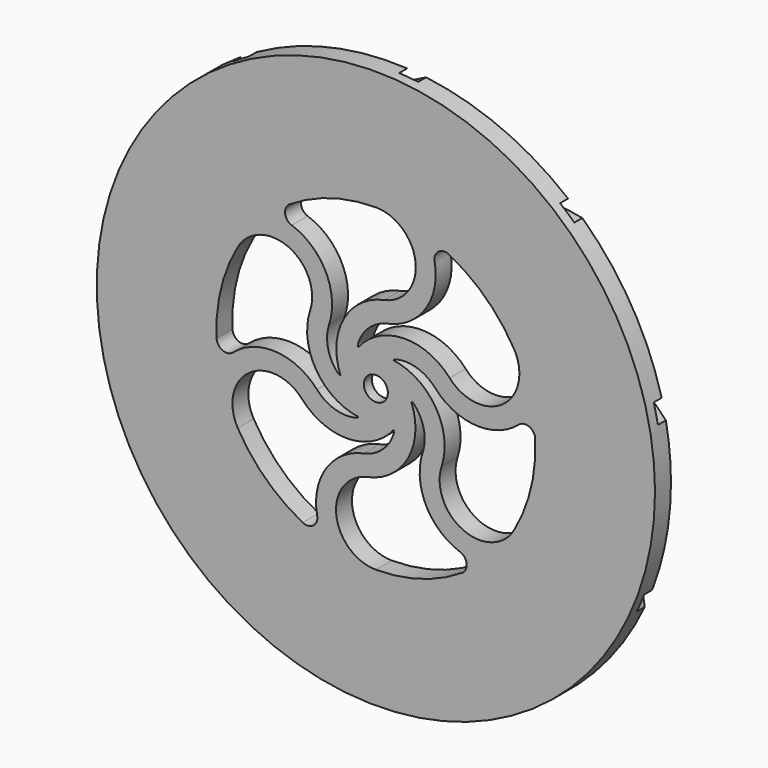
from build123d import *

# Parameters (mm, degrees)
F0_R           = 88.9
F1_DEPTH       = 6.35
F2_R           = 57.15
F2_R_2         = 53.975
F3_DEPTH       = 41.275
F5_DEPTH       = 41.275
F6_R           = 9.525
F6_R_2         = 3.81
F7_DEPTH       = 41.275
F8_R           = 3.81
F9_DEPTH       = 25.4
F10_R          = 2.54
F11_R          = 53.975
F12_DEPTH      = 41.2760001
F12_DEPTH_BACK = 3.175
F13_R          = 9.525
F13_R_2        = 3.81
F14_DEPTH      = 41.276
F14_DEPTH_BACK = 3.175


with BuildPart() as f1:
    # F0 (on Front) → F1 (new body)
    with BuildSketch(Plane.XZ):
        Circle(F0_R)
    extrude(amount=F1_DEPTH)

    # F2 (on face) → F3 (join)
    with BuildSketch(Plane.XZ.offset(6.35)):
        Circle(F2_R)
        Circle(F2_R_2, mode=Mode.SUBTRACT)
    extrude(amount=F3_DEPTH)

    # F4 (on face) → F5 (join, through all)
    with BuildSketch(Plane.XZ.offset(6.35)):
        with BuildLine():
            ThreePointArc((53.9069410952, -2.7096728137), (72.2551452316, -16.3352447412), (80.5410246247, -37.6344702686))
            ThreePointArc((80.5410246247, -37.6344702686), (81.7707619042, -34.8819795541), (82.9064652139, -32.0893755897))
            ThreePointArc((82.9064652139, -32.0893755897), (72.7373983183, -11.9238182989), (53.9711869017, 0.6415679441))
            ThreePointArc((53.9711869017, 0.6415679441), (53.9650843479, -1.0345512645), (53.9069410952, -2.7096728137))
        make_face()
        with BuildLine():
            ThreePointArc((45.2043371792, 29.4935336165), (68.0572563749, 29.2550181665), (87.2800442675, 16.8939004574))
            ThreePointArc((87.2800442675, 16.8939004574), (86.6570491761, 19.8435336593), (85.9344010285, 22.7703473815))
            ThreePointArc((85.9344010285, 22.7703473815), (65.8544359133, 33.10739838), (43.2865032341, 32.2425070794))
            ThreePointArc((43.2865032341, 32.2425070794), (44.2667643164, 30.8829111639), (45.2043371792, 29.4935336165))
        make_face()
        with BuildLine():
            ThreePointArc((19.2352128997, 50.4312126535), (37.863808764, 63.6708584761), (60.6810535397, 64.9693754112))
            ThreePointArc((60.6810535397, 64.9693754112), (58.4432890276, 66.9894914717), (56.1383164531, 68.9325715886))
            ThreePointArc((56.1383164531, 68.9325715886), (33.8173172993, 65.4927141568), (16.0678465853, 51.5279043928))
            ThreePointArc((16.0678465853, 51.5279043928), (17.6600448879, 51.0041511993), (19.2352128997, 50.4312126535))
        make_face()
        with BuildLine():
            ThreePointArc((-14.0811089267, 52.1058825508), (-6.7923268512, 73.7665949407), (10.9039628328, 88.2287571857))
            ThreePointArc((10.9039628328, 88.2287571857), (7.9061788848, 88.547740431), (4.8993030638, 88.7648963808))
            ThreePointArc((4.8993030638, 88.7648963808), (-11.1368671147, 72.8620391412), (-17.2881813331, 51.1313935972))
            ThreePointArc((-17.2881813331, 51.1313935972), (-15.6922114449, 51.6435390438), (-14.0811089267, 52.1058825508))
        make_face()
        with BuildLine():
            ThreePointArc((-42.0189257424, 33.8778763274), (-48.854024472, 55.6859993723), (-43.0380710641, 77.7877525005))
            ThreePointArc((-43.0380710641, 77.7877525005), (-45.6508228708, 76.2837621727), (-48.2110775747, 74.6920477634))
            ThreePointArc((-48.2110775747, 74.6920477634), (-51.837146819, 52.4005416633), (-44.0407115859, 31.2044283397))
            ThreePointArc((-44.0407115859, 31.2044283397), (-43.0505763644, 32.5568502729), (-42.0189257424, 33.8778763274))
        make_face()
        with BuildLine():
            ThreePointArc((-53.9069410952, 2.7096728137), (-72.2551452316, 16.3352447412), (-80.5410246247, 37.6344702686))
            ThreePointArc((-80.5410246247, 37.6344702686), (-81.7707619042, 34.8819795541), (-82.9064652139, 32.0893755897))
            ThreePointArc((-82.9064652139, 32.0893755897), (-72.7373983183, 11.9238182989), (-53.9711869017, -0.6415679441))
            ThreePointArc((-53.9711869017, -0.6415679441), (-53.9650843479, 1.0345512645), (-53.9069410952, 2.7096728137))
        make_face()
        with BuildLine():
            ThreePointArc((-45.2043371792, -29.4935336165), (-68.0572563749, -29.2550181665), (-87.2800442675, -16.8939004574))
            ThreePointArc((-87.2800442675, -16.8939004574), (-86.6570491761, -19.8435336593), (-85.9344010285, -22.7703473815))
            ThreePointArc((-85.9344010285, -22.7703473815), (-65.8544359133, -33.10739838), (-43.2865032341, -32.2425070794))
            ThreePointArc((-43.2865032341, -32.2425070794), (-44.2667643164, -30.8829111639), (-45.2043371792, -29.4935336165))
        make_face()
        with BuildLine():
            ThreePointArc((-19.2352128997, -50.4312126535), (-37.863808764, -63.6708584761), (-60.6810535397, -64.9693754112))
            ThreePointArc((-60.6810535397, -64.9693754112), (-58.4432890276, -66.9894914717), (-56.1383164531, -68.9325715886))
            ThreePointArc((-56.1383164531, -68.9325715886), (-33.8173172993, -65.4927141568), (-16.0678465853, -51.5279043928))
            ThreePointArc((-16.0678465853, -51.5279043928), (-17.6600448879, -51.0041511993), (-19.2352128997, -50.4312126535))
        make_face()
        with BuildLine():
            ThreePointArc((14.0811089267, -52.1058825508), (6.7923268512, -73.7665949407), (-10.9039628328, -88.2287571857))
            ThreePointArc((-10.9039628328, -88.2287571857), (-7.9061788848, -88.547740431), (-4.8993030638, -88.7648963808))
            ThreePointArc((-4.8993030638, -88.7648963808), (11.1368671147, -72.8620391412), (17.2881813331, -51.1313935972))
            ThreePointArc((17.2881813331, -51.1313935972), (15.6922114449, -51.6435390438), (14.0811089267, -52.1058825508))
        make_face()
        with BuildLine():
            ThreePointArc((42.0189257424, -33.8778763274), (48.854024472, -55.6859993723), (43.0380710641, -77.7877525005))
            ThreePointArc((43.0380710641, -77.7877525005), (45.6508228708, -76.2837621727), (48.2110775747, -74.6920477634))
            ThreePointArc((48.2110775747, -74.6920477634), (51.837146819, -52.4005416633), (44.0407115859, -31.2044283397))
            ThreePointArc((44.0407115859, -31.2044283397), (43.0505763644, -32.5568502729), (42.0189257424, -33.8778763274))
        make_face()
    extrude(amount=F5_DEPTH)

    # F6 (on face) → F7 (join, through all)
    with BuildSketch(Plane.XZ.offset(6.35)):
        Circle(F6_R)
        Circle(F6_R_2, mode=Mode.SUBTRACT)
    extrude(amount=F7_DEPTH)

    # F8 (on face) → F9 (cut)
    with BuildSketch(Plane.XZ.offset(6.35)):
        Circle(F8_R)
        with BuildLine():
            ThreePointArc((18.7012290876, 41.7285714286), (15.8576147996, 27.543553966), (3.8682590056, 19.446875))
            ThreePointArc((3.8682590056, 19.446875), (-2.091465664, 16.4126776534), (-5.6835018732, 10.7715831188))
            ThreePointArc((-5.6835018732, 10.7715831188), (-5.7538490333, 10.2503071963), (-5.6500021555, 9.7346589282))
            ThreePointArc((-5.6500021555, 9.7346589282), (8.7313709485, 16.9640191411), (23.5156008127, 10.5989512885))
            ThreePointArc((23.5156008127, 10.5989512885), (40.4349404037, 8.7570054641), (43.9940905122, 25.4))
            ThreePointArc((43.9940905122, 25.4), (35.0538695993, 36.7677334917), (23.2726406424, 45.1555555556))
            ThreePointArc((23.2726406424, 45.1555555556), (19.9136606493, 44.8737532722), (18.7012290876, 41.7285714286))
        make_face()
        with BuildLine():
            ThreePointArc((-11.2554630068, -0.025715934), (-10.3255860522, 16.0435986218), (2.5788393371, 25.6645833333))
            ThreePointArc((2.5788393371, 25.6645833333), (12.6336810088, 39.3961883222), (0, 50.8))
            ThreePointArc((0, 50.8), (-14.3148564437, 48.7414083198), (-27.4695379119, 42.7324757872))
            ThreePointArc((-27.4695379119, 42.7324757872), (-28.9049799722, 39.6826126407), (-26.787388377, 37.0600251862))
            ThreePointArc((-26.787388377, 37.0600251862), (-15.9246100453, 27.5048742428), (-14.9073582714, 13.0734480673))
            ThreePointArc((-14.9073582714, 13.0734480673), (-15.259528624, 6.3950764305), (-12.1702155565, 0.4637345547))
            ThreePointArc((-12.1702155565, 0.4637345547), (-11.7539509452, 0.1421741658), (-11.2554630068, -0.025715934))
        make_face()
        with BuildLine():
            ThreePointArc((-5.6054608513, -9.7603748622), (-19.0569570007, -0.9204205192), (-20.9367614757, 15.0656320448))
            ThreePointArc((-20.9367614757, 15.0656320448), (-27.8012593949, 30.6391828581), (-43.9940905122, 25.4))
            ThreePointArc((-43.9940905122, 25.4), (-49.368726043, 11.9736748281), (-50.7421785543, -2.4230797683))
            ThreePointArc((-50.7421785543, -2.4230797683), (-48.8186406215, -5.1911406315), (-45.4886174646, -4.6685462424))
            ThreePointArc((-45.4886174646, -4.6685462424), (-31.7822248448, -0.0386797232), (-18.775617277, -6.3734269327))
            ThreePointArc((-18.775617277, -6.3734269327), (-13.1680629599, -10.0176012229), (-6.4867136833, -10.3078485641))
            ThreePointArc((-6.4867136833, -10.3078485641), (-6.0001019119, -10.1081330305), (-5.6054608513, -9.7603748622))
        make_face()
        with BuildLine():
            ThreePointArc((5.6500021555, -9.7346589282), (-8.7313709485, -16.9640191411), (-23.5156008127, -10.5989512885))
            ThreePointArc((-23.5156008127, -10.5989512885), (-40.4349404037, -8.7570054641), (-43.9940905122, -25.4))
            ThreePointArc((-43.9940905122, -25.4), (-35.0538695993, -36.7677334917), (-23.2726406424, -45.1555555556))
            ThreePointArc((-23.2726406424, -45.1555555556), (-19.9136606493, -44.8737532722), (-18.7012290876, -41.7285714286))
            ThreePointArc((-18.7012290876, -41.7285714286), (-15.8576147996, -27.543553966), (-3.8682590056, -19.446875))
            ThreePointArc((-3.8682590056, -19.446875), (2.091465664, -16.4126776534), (5.6835018732, -10.7715831188))
            ThreePointArc((5.6835018732, -10.7715831188), (5.7538490333, -10.2503071963), (5.6500021555, -9.7346589282))
        make_face()
        with BuildLine():
            ThreePointArc((11.2554630068, 0.025715934), (10.3255860522, -16.0435986218), (-2.5788393371, -25.6645833333))
            ThreePointArc((-2.5788393371, -25.6645833333), (-12.6336810088, -39.3961883222), (0, -50.8))
            ThreePointArc((0, -50.8), (14.3148564437, -48.7414083198), (27.4695379119, -42.7324757872))
            ThreePointArc((27.4695379119, -42.7324757872), (28.9049799722, -39.6826126407), (26.787388377, -37.0600251862))
            ThreePointArc((26.787388377, -37.0600251862), (15.9246100453, -27.5048742428), (14.9073582714, -13.0734480673))
            ThreePointArc((14.9073582714, -13.0734480673), (15.259528624, -6.3950764305), (12.1702155565, -0.4637345547))
            ThreePointArc((12.1702155565, -0.4637345547), (11.7539509452, -0.1421741658), (11.2554630068, 0.025715934))
        make_face()
        with BuildLine():
            ThreePointArc((5.6054608513, 9.7603748622), (19.0569570007, 0.9204205192), (20.9367614757, -15.0656320448))
            ThreePointArc((20.9367614757, -15.0656320448), (27.8012593949, -30.6391828581), (43.9940905122, -25.4))
            ThreePointArc((43.9940905122, -25.4), (49.368726043, -11.9736748281), (50.7421785543, 2.4230797683))
            ThreePointArc((50.7421785543, 2.4230797683), (48.8186406215, 5.1911406315), (45.4886174646, 4.6685462424))
            ThreePointArc((45.4886174646, 4.6685462424), (31.7822248448, 0.0386797232), (18.775617277, 6.3734269327))
            ThreePointArc((18.775617277, 6.3734269327), (13.1680629599, 10.0176012229), (6.4867136833, 10.3078485641))
            ThreePointArc((6.4867136833, 10.3078485641), (6.0001019119, 10.1081330305), (5.6054608513, 9.7603748622))
        make_face()
    extrude(amount=-F9_DEPTH, mode=Mode.SUBTRACT)

    # F10
    f10_edges = [f1.edges().sort_by_distance(p)[0] for p in [
        (48.482356, -26.9875, 30.258613),
        (57.146896, -26.9875, -0.595661),
        (57.008616, -26.9875, -4.017481),
        (45.882689, -26.9875, -34.072002),
        (43.759523, -26.9875, -36.759035),
        (17.092855, -26.9875, -54.533997),
        (13.795779, -26.9875, -55.459886),
        (-18.225869, -26.9875, -54.165858),
        (-46.58293, -26.9875, -33.108203),
        (-21.437483, -26.9875, -52.976946),
        (-48.482356, -26.9875, -30.258613),
        (-57.008616, -26.9875, 4.017481),
        (-45.882689, -26.9875, 34.072002),
        (-57.146896, -26.9875, 0.595661),
        (-43.759523, -26.9875, 36.759035),
        (-17.092855, -26.9875, 54.533997),
        (-13.795779, -26.9875, 55.459886),
        (18.225869, -26.9875, 54.165858),
        (21.437483, -26.9875, 52.976946),
        (46.58293, -26.9875, 33.108203),
    ]]
    fillet(f10_edges, radius=F10_R)

    # F11 (on face) → F12 (cut, two sides)
    with BuildSketch(Plane.XZ.offset(6.35)) as f12_sk:
        with BuildLine():
            ThreePointArc((-10.9039628328, -88.2287571857), (-7.9061788848, -88.547740431), (-4.8993030638, -88.7648963808))
            ThreePointArc((-4.8993030638, -88.7648963808), (9.809736429, -74.9751556371), (16.9136887004, -56.1059570663))
            ThreePointArc((16.9136887004, -56.1059570663), (17.4652017585, -54.8309893719), (18.6049444803, -54.0368257847))
            ThreePointArc((18.6049444803, -54.0368257847), (30.8226195673, -48.1257584149), (41.3018706657, -39.5003541694))
            ThreePointArc((41.3018706657, -39.5003541694), (43.585469328, -38.755739099), (45.468484571, -40.2468890071))
            ThreePointArc((45.468484571, -40.2468890071), (48.7789098199, -59.3103123401), (43.0380710641, -77.7877525005))
            ThreePointArc((43.0380710641, -77.7877525005), (45.6508228708, -76.2837621727), (48.2110775747, -74.6920477634))
            ThreePointArc((48.2110775747, -74.6920477634), (52.0055342532, -54.8901566645), (46.6617157255, -35.4490559724))
            ThreePointArc((46.6617157255, -35.4490559724), (46.3584919542, -34.0934141983), (46.8137655409, -32.7809983966))
            ThreePointArc((46.8137655409, -32.7809983966), (53.2236340928, -20.8174752062), (56.6316409092, -7.6798273375))
            ThreePointArc((56.6316409092, -7.6798273375), (58.0414372783, -5.7351554754), (60.4413045354, -5.8347125026))
            ThreePointArc((60.4413045354, -5.8347125026), (74.3246939138, -19.3115268098), (80.5410246247, -37.6344702686))
            ThreePointArc((80.5410246247, -37.6344702686), (81.7707619042, -34.8819795541), (82.9064652139, -32.0893755897))
            ThreePointArc((82.9064652139, -32.0893755897), (74.3369855958, -13.8389834938), (58.5865533169, -1.2518203661))
            ThreePointArc((58.5865533169, -1.2518203661), (57.5444138906, -0.3333135935), (57.1413193063, 0.9960561938))
            ThreePointArc((57.1413193063, 0.9960561938), (55.2950293996, 14.4423759714), (50.330049164, 27.0741325096))
            ThreePointArc((50.330049164, 27.0741325096), (50.3275489442, 29.476062609), (52.3276004918, 30.8061258634))
            ThreePointArc((52.3276004918, 30.8061258634), (71.480971136, 28.0636055872), (87.2800442675, 16.8939004574))
            ThreePointArc((87.2800442675, 16.8939004574), (86.6570491761, 19.8435336593), (85.9344010285, 22.7703473815))
            ThreePointArc((85.9344010285, 22.7703473815), (68.274235062, 32.4982110017), (48.1333188249, 33.4235680723))
            ThreePointArc((48.1333188249, 33.4235680723), (46.7503255835, 33.5541014751), (45.6428312586, 34.3926511729))
            ThreePointArc((45.6428312586, 34.3926511729), (36.2456028847, 44.1857304062), (24.8040892936, 51.486693954))
            ThreePointArc((24.8040892936, 51.486693954), (23.3902474838, 53.4284266314), (24.2265316099, 55.6800712112))
            ThreePointArc((24.2265316099, 55.6800712112), (41.3339469332, 64.7193944968), (60.6810535397, 64.9693754112))
            ThreePointArc((60.6810535397, 64.9693754112), (58.4432890276, 66.9894914717), (56.1383164531, 68.9325715886))
            ThreePointArc((56.1383164531, 68.9325715886), (36.1330472904, 66.4221934682), (19.2947925332, 55.3322895323))
            ThreePointArc((19.2947925332, 55.3322895323), (18.0992018886, 54.6249902422), (16.710333013, 54.6524223671))
            ThreePointArc((16.710333013, 54.6524223671), (3.3515880106, 57.0516376435), (-10.1961896269, 56.2330882763))
            ThreePointArc((-10.1961896269, 56.2330882763), (-12.4813335101, 56.972947646), (-13.1282489173, 59.2861218524))
            ThreePointArc((-13.1282489173, 59.2861218524), (-4.601240109, 76.6545744399), (10.9039628328, 88.2287571857))
            ThreePointArc((10.9039628328, 88.2287571857), (7.9061788848, 88.547740431), (4.8993030638, 88.7648963808))
            ThreePointArc((4.8993030638, 88.7648963808), (-9.809736429, 74.9751556371), (-16.9136887004, 56.1059570663))
            ThreePointArc((-16.9136887004, 56.1059570663), (-17.4652017585, 54.8309893719), (-18.6049444803, 54.0368257847))
            ThreePointArc((-18.6049444803, 54.0368257847), (-30.8226195673, 48.1257584149), (-41.3018706657, 39.5003541694))
            ThreePointArc((-41.3018706657, 39.5003541694), (-43.585469328, 38.755739099), (-45.468484571, 40.2468890071))
            ThreePointArc((-45.468484571, 40.2468890071), (-48.7789098199, 59.3103123401), (-43.0380710641, 77.7877525005))
            ThreePointArc((-43.0380710641, 77.7877525005), (-45.6508228708, 76.2837621727), (-48.2110775747, 74.6920477634))
            ThreePointArc((-48.2110775747, 74.6920477634), (-52.0055342532, 54.8901566645), (-46.6617157255, 35.4490559724))
            ThreePointArc((-46.6617157255, 35.4490559724), (-46.3584919542, 34.0934141983), (-46.8137655409, 32.7809983966))
            ThreePointArc((-46.8137655409, 32.7809983966), (-53.2236340928, 20.8174752062), (-56.6316409092, 7.6798273375))
            ThreePointArc((-56.6316409092, 7.6798273375), (-58.0414372783, 5.7351554754), (-60.4413045354, 5.8347125026))
            ThreePointArc((-60.4413045354, 5.8347125026), (-74.3246939138, 19.3115268098), (-80.5410246247, 37.6344702686))
            ThreePointArc((-80.5410246247, 37.6344702686), (-81.7707619042, 34.8819795541), (-82.9064652139, 32.0893755897))
            ThreePointArc((-82.9064652139, 32.0893755897), (-74.3369855958, 13.8389834938), (-58.5865533169, 1.2518203661))
            ThreePointArc((-58.5865533169, 1.2518203661), (-57.5444138906, 0.3333135935), (-57.1413193063, -0.9960561938))
            ThreePointArc((-57.1413193063, -0.9960561938), (-55.2950293996, -14.4423759714), (-50.330049164, -27.0741325096))
            ThreePointArc((-50.330049164, -27.0741325096), (-50.3275489442, -29.476062609), (-52.3276004918, -30.8061258634))
            ThreePointArc((-52.3276004918, -30.8061258634), (-71.480971136, -28.0636055872), (-87.2800442675, -16.8939004574))
            ThreePointArc((-87.2800442675, -16.8939004574), (-86.6570491761, -19.8435336593), (-85.9344010285, -22.7703473815))
            ThreePointArc((-85.9344010285, -22.7703473815), (-68.274235062, -32.4982110017), (-48.1333188249, -33.4235680723))
            ThreePointArc((-48.1333188249, -33.4235680723), (-46.7503255835, -33.5541014751), (-45.6428312586, -34.3926511729))
            ThreePointArc((-45.6428312586, -34.3926511729), (-36.2456028847, -44.1857304062), (-24.8040892936, -51.486693954))
            ThreePointArc((-24.8040892936, -51.486693954), (-23.3902474838, -53.4284266314), (-24.2265316099, -55.6800712112))
            ThreePointArc((-24.2265316099, -55.6800712112), (-41.3339469332, -64.7193944968), (-60.6810535397, -64.9693754112))
            ThreePointArc((-60.6810535397, -64.9693754112), (-58.4432890276, -66.9894914717), (-56.1383164531, -68.9325715886))
            ThreePointArc((-56.1383164531, -68.9325715886), (-36.1330472904, -66.4221934682), (-19.2947925332, -55.3322895323))
            ThreePointArc((-19.2947925332, -55.3322895323), (-18.0992018886, -54.6249902422), (-16.710333013, -54.6524223671))
            ThreePointArc((-16.710333013, -54.6524223671), (-3.3515880106, -57.0516376435), (10.1961896269, -56.2330882763))
            ThreePointArc((10.1961896269, -56.2330882763), (12.4813335101, -56.972947646), (13.1282489173, -59.2861218524))
            ThreePointArc((13.1282489173, -59.2861218524), (4.601240109, -76.6545744399), (-10.9039628328, -88.2287571857))
        make_face()
        Circle(F11_R, mode=Mode.SUBTRACT)
    extrude(amount=F12_DEPTH, mode=Mode.SUBTRACT)
    extrude(f12_sk.sketch, amount=-F12_DEPTH_BACK, mode=Mode.SUBTRACT)

    # F13 (on face) → F14 (cut, two sides)
    with BuildSketch(Plane.XZ.offset(6.35)) as f14_sk:
        Circle(F13_R)
        Circle(F13_R_2, mode=Mode.SUBTRACT)
    extrude(amount=F14_DEPTH, mode=Mode.SUBTRACT)
    extrude(f14_sk.sketch, amount=-F14_DEPTH_BACK, mode=Mode.SUBTRACT)


with BuildPart() as f16_1:
    # F16: instance of F1
    add(f1.part.mirror(Plane.XZ.offset(25.4)))


solid = f16_1.part
